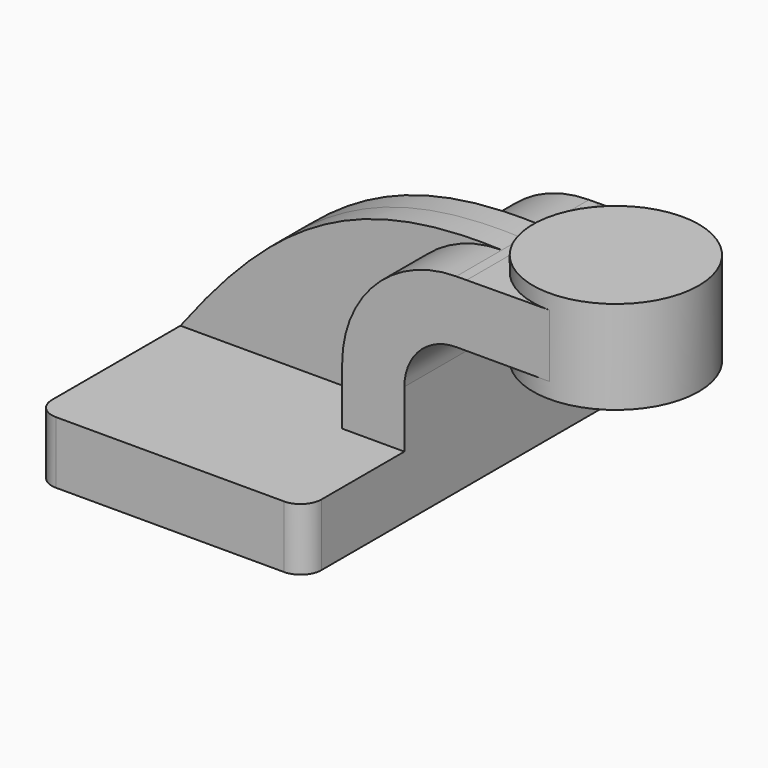
from build123d import *

# Parameters (mm, degrees)
F1_DEPTH = 63.5
F2_DEPTH = 25.4
F3_DEPTH = 7.9375
F0_W     = 25.4
F0_H     = 4.7752
F5_R     = 6.35


with BuildPart() as f1:
    # F0 (on Front) → F1 (new body, symmetric)
    with BuildSketch(Plane.XZ):
        Polygon((22.225, 9.525), (-41.275, 9.525), (-41.275, -9.525), (41.275, -9.525), (41.275, 9.525), align=None)
    extrude(amount=F1_DEPTH, both=True)

    # F0 (on Front) → F2 (join, symmetric)
    with BuildSketch(Plane.XZ):
        with BuildLine():
            Line((22.225, 27.0002), (22.225, 9.525))
            Line((22.225, 9.525), (41.275, 9.525))
            Line((41.275, 9.525), (41.275, 27.0002))
            ThreePointArc((41.275, 27.0002), (45.9246798487, 38.2255201513), (57.15, 42.8752))
            Line((57.15, 42.8752), (60.325, 42.8752))
            Line((60.325, 42.8752), (60.325, 61.9476745522))
            Line((60.325, 61.9476745522), (57.15, 61.9252))
            ThreePointArc((57.15, 61.9252), (32.4542956671, 51.6959043329), (22.225, 27.0002))
        make_face()
        Polygon((85.725, 62.1274709702), (60.325, 61.9476745522), (60.325, 42.8752), (85.725, 42.8752), align=None)
    extrude(amount=F2_DEPTH, both=True)

    # F0 (on Front) → F3 (join, symmetric)
    with BuildSketch(Plane.XZ):
        with BuildLine():
            add(Edge.make_bspline(
                [(-41.275, 9.525), (-12.9327131435, 46.9444841146), (11.8099329993, 63.8144686818), (57.15, 61.9252)],
                knots=[0, 0, 0, 0, 111.5045361635, 111.5045361635, 111.5045361635, 111.5045361635], degree=3))
            Line((-41.275, 9.525), (22.225, 9.525))
            Line((22.225, 9.525), (22.225, 27.0002))
            ThreePointArc((22.225, 27.0002), (32.4542956671, 51.6959043329), (57.15, 61.9252))
        make_face()
    extrude(amount=F3_DEPTH, both=True)

    # F0 (on Front) → F4 (revolve)
    with BuildSketch(Plane.XZ):
        Polygon((85.725, 66.675), (85.725, 62.1274709702), (85.725, 42.8752), (111.125, 42.8752), (111.125, 66.675), align=None)
        with Locations((98.425, 40.4876)):
            Rectangle(F0_W, F0_H)
    revolve(axis=Axis((85.725, 0, 52.3875), (0, 0, 1)))

    # F5
    f5_edges = [f1.edges().sort_by_distance(p)[0] for p in [
        (-41.275, -63.5, 0),
        (41.275, -63.5, 0),
        (41.275, 63.5, 0),
        (-41.275, 63.5, 0),
    ]]
    fillet(f5_edges, radius=F5_R)


solid = f1.part
